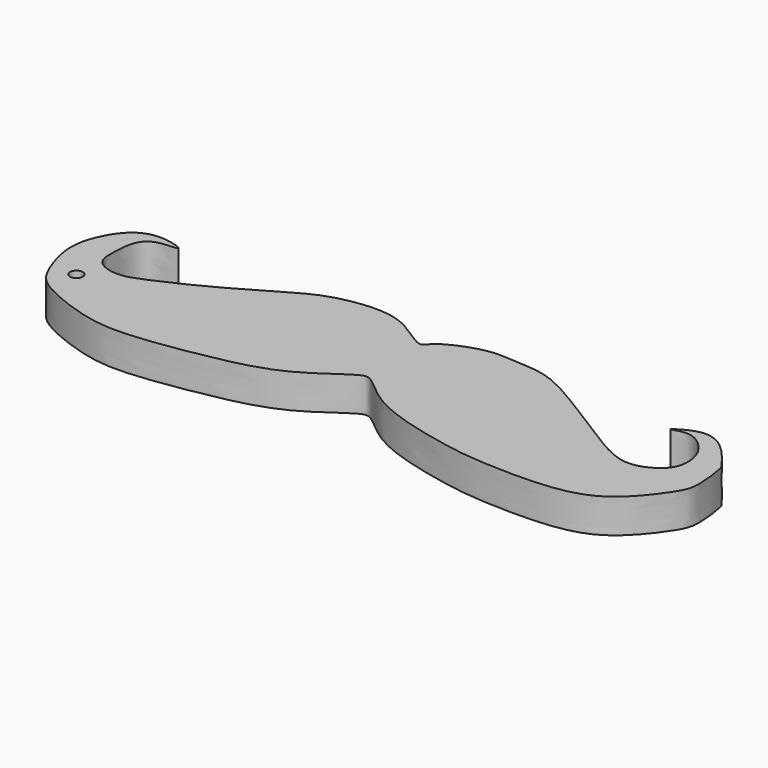
from build123d import *

# Parameters (mm, degrees)
F1_DEPTH = 8
F3_D     = 3


with BuildPart() as f1:
    # F0 (on Top) → F1 (new body)
    with BuildSketch(Plane.XY):
        with BuildLine():
            add(Edge.make_bspline(
                [(-75.6464749575, 31.5007641912), (-76.7966589362, 31.462026151), (-81.9548146192, 35.5916384526), (-88.9054688558, 38.0292874739), (-100.6190798464, 36.4909187751), (-108.7328494702, 31.6979440455), (-120.623254768, 24.7208767874), (-130.5500378611, 20.2025704515), (-136.2705427081, 17.8994315243), (-142.431680229, 19.8949321546), (-142.362330017, 24.9486516384), (-142.1861605977, 29.6492046846), (-139.722485578, 33.5597066786), (-131.4461446901, 33.0271560961), (-139.19512761, 35.6093272707), (-145.5199808584, 33.6159595594), (-149.6308455561, 25.8412697276), (-150.0960729966, 19.2559354372), (-147.0562544505, 10.5184794468), (-143.2842426172, 6.3720829266), (-130.2824961178, 1.2175083732), (-119.9084711824, 0.5591322166), (-102.0321857293, 3.397399549), (-87.48956966, 6.844444372), (-77.2626693707, 15.20123863), (-74.0212509497, 15.6593788114), (-66.8470501567, 7.4984416295), (-48.0191703565, 3.2793185003), (-39.8569836613, 1.9835394845), (-25.0885947343, 1.4555073152), (-11.1413984618, 3.4418841805), (-2.6959124257, 14.6874634023), (-0.5989347386, 18.9232109666), (-1.8871935251, 27.6398129777), (-2.5288898174, 28.3476202881), (-7.7389725115, 35.616505154), (-14.0185667704, 37.2621393992), (-20.7758409974, 32.6846106915), (-14.7269125857, 35.50050368), (-9.9286833775, 31.5494858828), (-8.031556564, 27.3869011129), (-8.2363407898, 21.9790892795), (-13.5694173047, 18.4661595051), (-19.8767170856, 18.0610972076), (-31.1388262684, 25.7291713392), (-36.9499521701, 29.0651586894), (-49.4006891202, 37.1313938649), (-57.7335421156, 36.7828455991), (-64.2867934472, 37.9597844856), (-74.2822404333, 33.6799117903), (-74.9873294321, 31.5229641229), (-75.6464749575, 31.5007641912)],
                knots=[0, 0, 0, 0, 0.0189971268, 0.0395955118, 0.0638747696, 0.0865537716, 0.1137466455, 0.1379746968, 0.1558828915, 0.1726215724, 0.1879574754, 0.2038439643, 0.2191107552, 0.2351909725, 0.2507158869, 0.269829091, 0.290562263, 0.3095258305, 0.3310105601, 0.3483007938, 0.3747410382, 0.3988661045, 0.4294980637, 0.4587374145, 0.4841852206, 0.4955060337, 0.5183958741, 0.5503519566, 0.5719640318, 0.5994779205, 0.6269685886, 0.6530091331, 0.6696727519, 0.6901274286, 0.6980389533, 0.7188467312, 0.737983464, 0.7538618339, 0.7674055009, 0.7852095849, 0.8008232037, 0.8168295449, 0.8341647171, 0.8521649116, 0.8783332312, 0.8984995125, 0.9259058432, 0.9466581047, 0.9657501929, 0.9891131581, 1, 1, 1, 1], degree=3))
        make_face()
    extrude(amount=F1_DEPTH)

    # F3 (through all)
    with Locations(Plane.XY.offset(8)):
        with Locations((-142.1997398138, 13.7817617506)):
            Hole(F3_D / 2)


solid = f1.part
